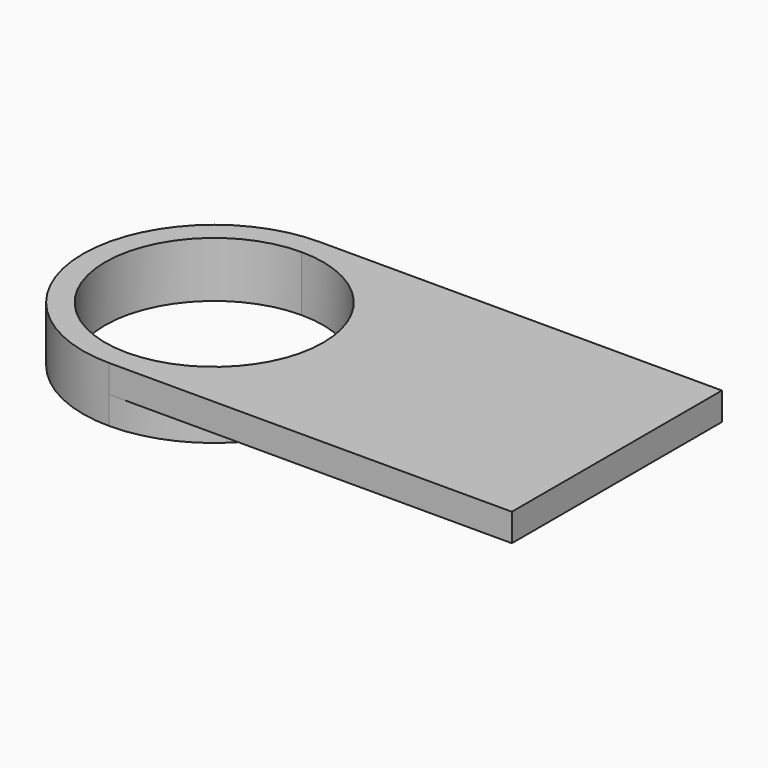
from build123d import *

# Parameters (mm, degrees)
F1_DEPTH = 101.6
F2_DEPTH = 101.6


with BuildPart() as f1:
    # F0 (on Top) → F1 (new body)
    with BuildSketch(Plane.XY):
        with BuildLine():
            ThreePointArc((-737.234056, 480.760509), (-1217.994565, 0), (-737.234056, -480.760509))
            Line((-737.234056, -480.760509), (-737.234056, -399.259402))
            ThreePointArc((-737.234056, -399.259402), (-1136.493458, 0), (-737.234056, 399.259402))
            Line((-737.234056, 399.259402), (-737.234056, 480.760509))
        make_face()
        with BuildLine():
            Line((-737.234056, -399.259402), (-737.234056, -480.760509))
            ThreePointArc((-737.234056, -480.760509), (-397.28504, -339.949016), (-256.473547, 0))
            ThreePointArc((-256.473547, 0), (-397.28504, 339.949016), (-737.234056, 480.760509))
            Line((-737.234056, 480.760509), (-737.234056, 399.259402))
            ThreePointArc((-737.234056, 399.259402), (-454.915025, 282.319031), (-337.974654, 0))
            ThreePointArc((-337.974654, 0), (-454.915025, -282.319031), (-737.234056, -399.259402))
        make_face()
        with BuildLine():
            Line((-737.234056, -480.760509), (737.234056, -480.760509))
            Line((737.234056, -480.760509), (737.234056, 480.760509))
            Line((737.234056, 480.760509), (-737.234056, 480.760509))
            ThreePointArc((-737.234056, 480.760509), (-397.28504, 339.949016), (-256.473547, 0))
            ThreePointArc((-256.473547, 0), (-397.28504, -339.949016), (-737.234056, -480.760509))
        make_face()
    extrude(amount=F1_DEPTH)

    # F0 (on Top) → F2 (join)
    with BuildSketch(Plane.XY):
        with BuildLine():
            Line((-737.234056, -399.259402), (-737.234056, -480.760509))
            ThreePointArc((-737.234056, -480.760509), (-397.28504, -339.949016), (-256.473547, 0))
            ThreePointArc((-256.473547, 0), (-397.28504, 339.949016), (-737.234056, 480.760509))
            Line((-737.234056, 480.760509), (-737.234056, 399.259402))
            ThreePointArc((-737.234056, 399.259402), (-454.915025, 282.319031), (-337.974654, 0))
            ThreePointArc((-337.974654, 0), (-454.915025, -282.319031), (-737.234056, -399.259402))
        make_face()
        with BuildLine():
            ThreePointArc((-737.234056, 480.760509), (-1217.994565, 0), (-737.234056, -480.760509))
            Line((-737.234056, -480.760509), (-737.234056, -399.259402))
            ThreePointArc((-737.234056, -399.259402), (-1136.493458, 0), (-737.234056, 399.259402))
            Line((-737.234056, 399.259402), (-737.234056, 480.760509))
        make_face()
    extrude(amount=-F2_DEPTH)


solid = f1.part
